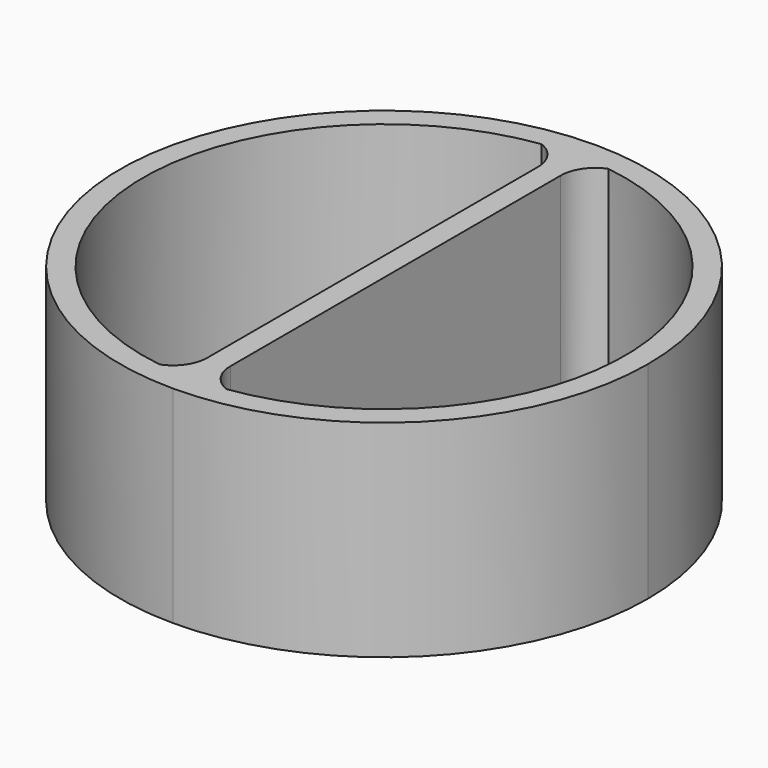
from build123d import *

# Parameters (mm, degrees)
F1_DEPTH = 57.15
F2_DEPTH = 3.175


# Not quite as in the source:
# - a feature names something its author has since deleted; it is built from what else it names


with BuildPart() as f1:
    # F0 (on Top) → F1 (new body)
    with BuildSketch(Plane.XY):
        with BuildLine():
            ThreePointArc((0, -73.025), (51.6364726961, -51.6364726961), (73.025, 0))
            ThreePointArc((73.025, 0), (51.6364726961, 51.6364726961), (0, 73.025))
            Line((0, 73.025), (0, 66.675))
            ThreePointArc((0, 66.675), (1.5879504187, 66.6560877825), (3.175, 66.5993618588))
            ThreePointArc((3.175, 66.5993618588), (6.220920948, 66.3841529852), (9.2537943589, 66.0297123647))
            ThreePointArc((9.2537943589, 66.0297123647), (50.3117896913, 43.752479279), (66.675, 0))
            ThreePointArc((66.675, 0), (50.3117896913, -43.752479279), (9.2537943589, -66.0297123647))
            ThreePointArc((9.2537943589, -66.0297123647), (6.220920948, -66.3841529852), (3.175, -66.5993618588))
            ThreePointArc((3.175, -66.5993618588), (1.5879504187, -66.6560877825), (0, -66.675))
            Line((0, -66.675), (0, -73.025))
        make_face()
        with BuildLine():
            Line((0, 66.675), (0, 73.025))
            ThreePointArc((0, 73.025), (-73.025, 0), (0, -73.025))
            Line((0, -73.025), (0, -66.675))
            ThreePointArc((0, -66.675), (-1.5879504187, -66.6560877825), (-3.175, -66.5993618588))
            ThreePointArc((-3.175, -66.5993618588), (-6.220920948, -66.3841529852), (-9.2537943589, -66.0297123647))
            ThreePointArc((-9.2537943589, -66.0297123647), (-66.675, 0), (-9.2537943589, 66.0297123647))
            ThreePointArc((-9.2537943589, 66.0297123647), (-6.220920948, 66.3841529852), (-3.175, 66.5993618588))
            ThreePointArc((-3.175, 66.5993618588), (-1.5879504187, 66.6560877825), (0, 66.675))
        make_face()
        with BuildLine():
            Line((-3.175, 57.15), (-3.175, 66.5993618588))
            ThreePointArc((-3.175, 66.5993618588), (-6.220920948, 66.3841529852), (-9.2537943589, 66.0297123647))
            ThreePointArc((-9.2537943589, 66.0297123647), (-4.840269288, 62.5305444087), (-3.175, 57.15))
        make_face()
        with BuildLine():
            ThreePointArc((9.2537943589, 66.0297123647), (6.220920948, 66.3841529852), (3.175, 66.5993618588))
            Line((3.175, 66.5993618588), (3.175, 57.15))
            ThreePointArc((3.175, 57.15), (4.840269288, 62.5305444087), (9.2537943589, 66.0297123647))
        make_face()
        with BuildLine():
            Line((3.175, -57.15), (3.175, -66.5993618588))
            ThreePointArc((3.175, -66.5993618588), (6.220920948, -66.3841529852), (9.2537943589, -66.0297123647))
            ThreePointArc((9.2537943589, -66.0297123647), (4.840269288, -62.5305444087), (3.175, -57.15))
        make_face()
        with BuildLine():
            ThreePointArc((-9.2537943589, -66.0297123647), (-6.220920948, -66.3841529852), (-3.175, -66.5993618588))
            Line((-3.175, -66.5993618588), (-3.175, -57.15))
            ThreePointArc((-3.175, -57.15), (-4.840269288, -62.5305444087), (-9.2537943589, -66.0297123647))
        make_face()
        with BuildLine():
            Line((0, -66.675), (0, 66.675))
            ThreePointArc((0, 66.675), (-1.5879504187, 66.6560877825), (-3.175, 66.5993618588))
            Line((-3.175, 66.5993618588), (-3.175, 57.15))
            Line((-3.175, 57.15), (-3.175, -57.15))
            Line((-3.175, -57.15), (-3.175, -66.5993618588))
            ThreePointArc((-3.175, -66.5993618588), (-1.5879504187, -66.6560877825), (0, -66.675))
        make_face()
        with BuildLine():
            ThreePointArc((3.175, 66.5993618588), (1.5879504187, 66.6560877825), (0, 66.675))
            Line((0, 66.675), (0, -66.675))
            ThreePointArc((0, -66.675), (1.5879504187, -66.6560877825), (3.175, -66.5993618588))
            Line((3.175, -66.5993618588), (3.175, -57.15))
            Line((3.175, -57.15), (3.175, 57.15))
            Line((3.175, 57.15), (3.175, 66.5993618588))
        make_face()
    extrude(amount=F1_DEPTH)

    # F0 (on Top) → F2 (join)
    with BuildSketch(Plane.XY):
        with BuildLine():
            ThreePointArc((-3.175, 57.15), (-4.840269288, 62.5305444087), (-9.2537943589, 66.0297123647))
            ThreePointArc((-9.2537943589, 66.0297123647), (-66.675, 0), (-9.2537943589, -66.0297123647))
            ThreePointArc((-9.2537943589, -66.0297123647), (-4.840269288, -62.5305444087), (-3.175, -57.15))
            Line((-3.175, -57.15), (-3.175, 57.15))
        make_face()
        with BuildLine():
            ThreePointArc((66.675, 0), (50.3117896913, 43.752479279), (9.2537943589, 66.0297123647))
            ThreePointArc((9.2537943589, 66.0297123647), (4.840269288, 62.5305444087), (3.175, 57.15))
            Line((3.175, 57.15), (3.175, -57.15))
            ThreePointArc((3.175, -57.15), (4.840269288, -62.5305444087), (9.2537943589, -66.0297123647))
            ThreePointArc((9.2537943589, -66.0297123647), (50.3117896913, -43.752479279), (66.675, 0))
        make_face()
    extrude(amount=F2_DEPTH)


solid = f1.part
